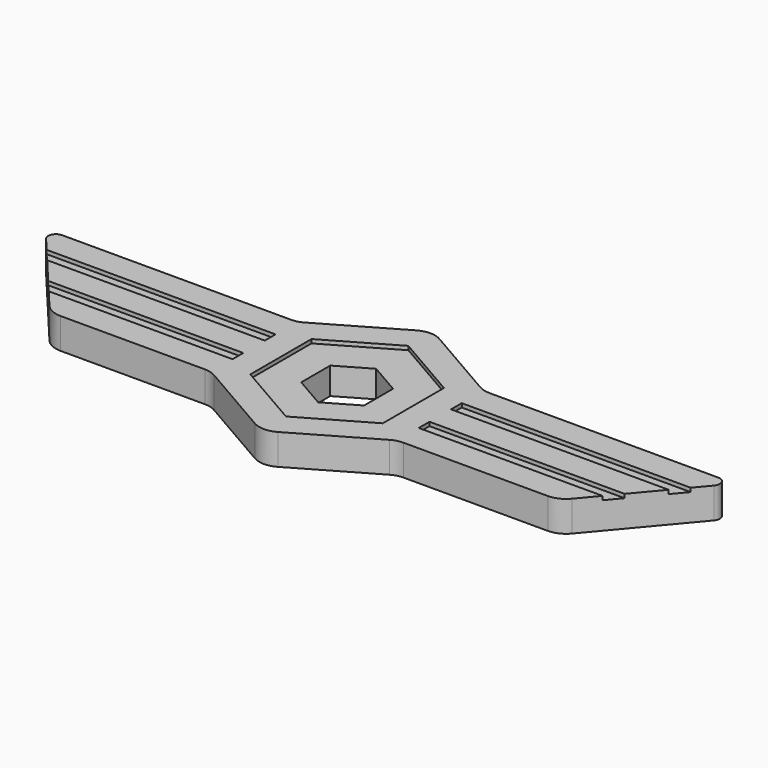
from build123d import *

# Parameters (mm, degrees)
F1_DEPTH = 4
F2_R     = 1
F3_R     = 3
F5_DEPTH = 0.5


with BuildPart() as f1:
    # F0 (on Top) → F1 (new body)
    with BuildSketch(Plane.XY):
        Polygon((-12.124355653, 7), (-30.1414284285, 7), (-44.8717504895, 7), (-33.124355653, -7), (-12.124355653, -7), (0, -14), (12.124355653, -7), (33.124355653, -7), (44.8717504895, 7), (30.1414284285, 7), (12.124355653, 7), (0, 14), align=None)
        Polygon((4.09, 2.361362601), (4.09, -2.361362601), (0, -4.722725202), (-4.09, -2.361362601), (-4.09, 2.361362601), (0, 4.722725202), align=None, mode=Mode.SUBTRACT)
    extrude(amount=F1_DEPTH)

    # F2
    f2_edges = [f1.edges().sort_by_distance(p)[0] for p in [
        (-44.87175, 7, 2),
        (44.87175, 7, 2),
    ]]
    fillet(f2_edges, radius=F2_R)

    # F3
    f3_edges = [f1.edges().sort_by_distance(p)[0] for p in [
        (-33.124356, -7, 2),
        (-12.124356, -7, 2),
        (12.124356, -7, 2),
        (12.124356, 7, 2),
        (-12.124356, 7, 2),
        (0, -14, 2),
        (0, 14, 2),
        (33.124356, -7, 2),
    ]]
    fillet(f3_edges, radius=F3_R)

    # F4 (on face) → F5 (cut)
    with BuildSketch(Plane.XY.offset(4)):
        Polygon((0, -9.9585481157), (8.624355653, -4.9792740578), (8.624355653, 4.9792740578), (0, 9.9585481157), (-8.624355653, 4.9792740578), (-8.624355653, -4.9792740578), align=None)
        Polygon((4.09, 2.361362601), (4.09, -2.361362601), (0, -4.722725202), (-4.09, -2.361362601), (-4.09, 2.361362601), (0, 4.722725202), align=None, mode=Mode.SUBTRACT)
        Polygon((-12.124355653, 3.5), (-41.9349017803, 3.5), (-40.4664774258, 1.75), (-12.124355653, 1.75), align=None)
        Polygon((-12.124355653, -1.75), (-37.5296287167, -1.75), (-36.0612043621, -3.5), (-12.124355653, -3.5), align=None)
        Polygon((12.124355653, 3.5), (12.124355653, 1.75), (40.4664774258, 1.75), (41.9349017803, 3.5), align=None)
        Polygon((36.0612043621, -3.5), (37.5296287167, -1.75), (12.124355653, -1.75), (12.124355653, -3.5), align=None)
    extrude(amount=-F5_DEPTH, mode=Mode.SUBTRACT)


solid = f1.part
